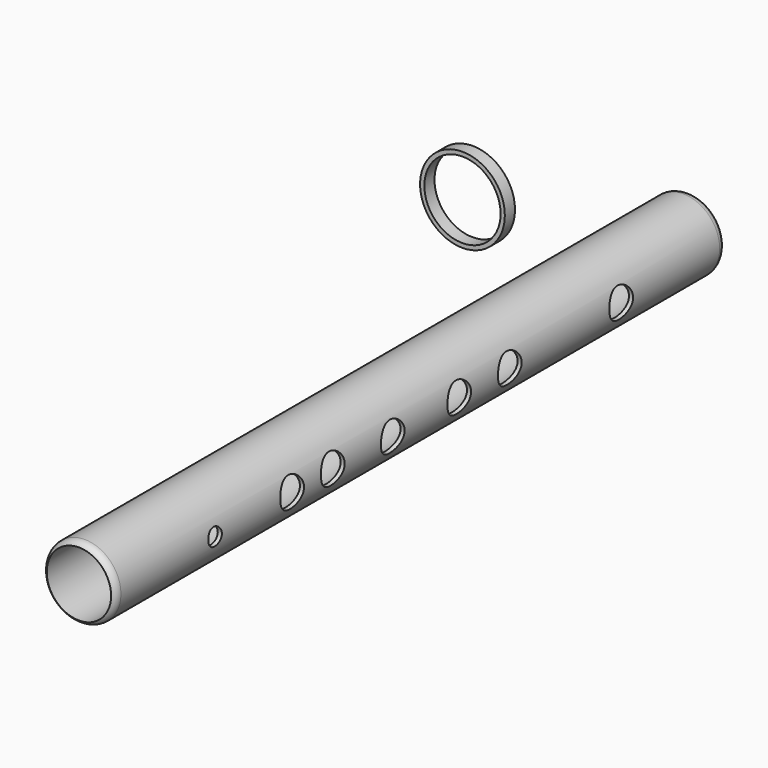
from build123d import *

# Parameters (mm, degrees)
F0_R      = 21.7516841919
F1_DEPTH  = 457.2
F3_R      = 25.4
F4_DEPTH  = 7.62
F5_R      = 22.86
F6_DEPTH  = 7.621
F7_R      = 8.89
F7_R_2    = 5.08
F8_DEPTH  = 184.8046559513
F9_R      = 19.2907082919
F10_DEPTH = 457.2010001


# Not quite as in the source:
# - a fillet or chamfer that OpenCascade refuses, or shapes differently, is made with other operations: its cross-section is extruded or revolved along the edge and cut away or added


with BuildPart() as f1:
    # F0 (on Front) → F1 (new body)
    with BuildSketch(Plane.XZ):
        with Locations((-29.6561513096, 11.0696014017)):
            Circle(F0_R)
    extrude(amount=F1_DEPTH)

    # F7 (on Right) → F8 (cut, through all)
    with BuildSketch(Plane.YZ):
        with Locations((-78.0123621225, 11.8408035487)):
            Circle(F7_R)
        with Locations((-161.4900231361, 11.2487627193)):
            Circle(F7_R)
        with Locations((-199.3806064129, 11.2487627193)):
            Circle(F7_R)
        with Locations((-249.1924315691, 10.8174476773)):
            Circle(F7_R)
        with Locations((-294.1070199013, 12.0607232675)):
            Circle(F7_R)
        with Locations((-324.5849609375, 12.0607232675)):
            Circle(F7_R)
        with Locations((-382.3210000992, 12.4328434467)):
            Circle(F7_R_2)
    extrude(amount=-F8_DEPTH, mode=Mode.SUBTRACT)

    # F9 (on face) → F10 (cut, through all)
    with BuildSketch(Plane(origin=(0, 0, 0), x_dir=(-1, 0, 0), z_dir=(0, 1, 0))):
        with Locations((29.6561513096, 11.0696014017)):
            Circle(F9_R)
    extrude(amount=-F10_DEPTH, mode=Mode.SUBTRACT)

    # F11: fillet of radius 5.08 on 1 edges, made by hand

    # F11_s1 → F11_t2 (revolve, cut)
    with BuildSketch(Plane.XY.offset(11.0696014017)):
        with BuildLine():
            ThreePointArc((-7.9040671177, -4.3533740732), (-8.5619471018, -1.8527638517), (-10.3652367585, 0.0003427202))
            Line((-10.3652367585, 0.0003427202), (-10.103217154, 0.4357143995))
            ThreePointArc((-10.103217154, 0.4357143995), (-9.1348519381, 0.5081365685), (-7.9044671177, 0.5081365685))
            Line((-7.9044671177, 0.5081365685), (-7.3963305491, 0))
            ThreePointArc((-7.3963305491, 0), (-7.3963305491, -2.1766870366), (-7.3959305491, -4.3533740732))
            Line((-7.3959305491, -4.3533740732), (-7.9040671177, -4.3533740732))
        make_face()
    revolve(axis=Axis((-29.6561513096, 0, 11.0696014017), (0, -1, 0)), mode=Mode.SUBTRACT)

    # F12: fillet of radius 5.08 on 1 edges, made by hand

    # F12_s1 → F12_t2 (revolve, cut)
    with BuildSketch(Plane.XY.offset(11.0696014017)):
        with BuildLine():
            ThreePointArc((-7.9040671177, -452.8466259268), (-8.5619471018, -455.3472361483), (-10.3652367585, -457.2003427202))
            Line((-10.3652367585, -457.2003427202), (-10.103217154, -457.6357143995))
            ThreePointArc((-10.103217154, -457.6357143995), (-9.1348519381, -457.7081365685), (-7.9044671177, -457.7081365685))
            Line((-7.9044671177, -457.7081365685), (-7.3963305491, -457.2))
            ThreePointArc((-7.3963305491, -457.2), (-7.3963305491, -455.0233129634), (-7.3959305491, -452.8466259268))
            Line((-7.3959305491, -452.8466259268), (-7.9040671177, -452.8466259268))
        make_face()
    revolve(axis=Axis((-29.6561513096, -457.2, 11.0696014017), (0, -1, 0)), mode=Mode.SUBTRACT)


with BuildPart() as f4:
    # F3 (on Front) → F4 (new body)
    with BuildSketch(Plane.XZ):
        with Locations((-159.4036559513, -11.164822271)):
            Circle(F3_R)
    extrude(amount=F4_DEPTH)

    # F5 (on face) → F6 (cut, through all)
    with BuildSketch(Plane.XZ.offset(7.62)):
        with Locations((-159.4036559513, -11.164822271)):
            Circle(F5_R)
    extrude(amount=-F6_DEPTH, mode=Mode.SUBTRACT)


solid = Compound([f1.part, f4.part])
